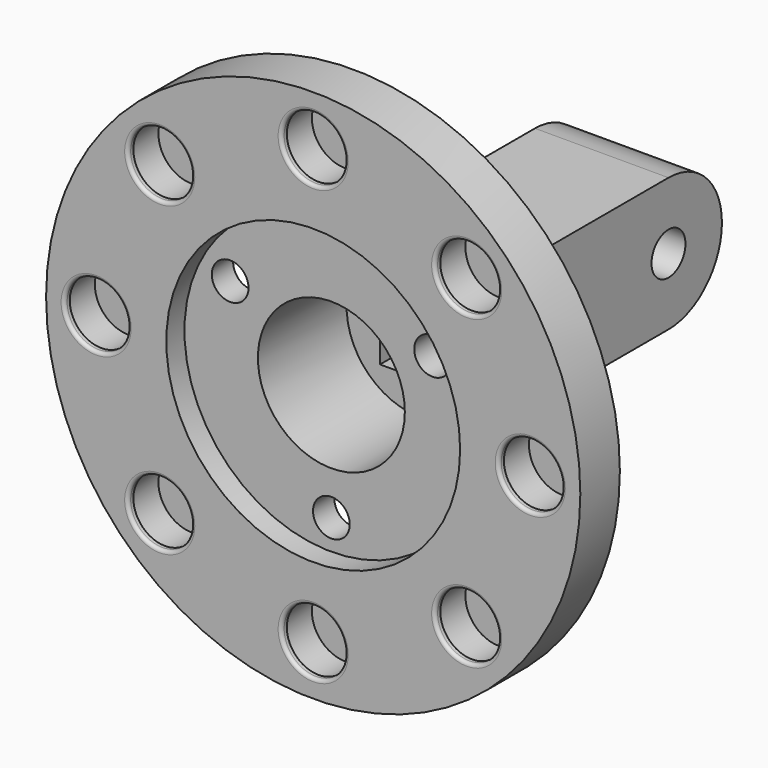
from build123d import *

# Parameters (mm, degrees)
F0_W      = 20
F0_H      = 30
F1_DEPTH  = 20
F2_R      = 9.99999
F3_R      = 3.175
F4_DEPTH  = 25
F5_DEPTH  = 10
F6_T      = -4
F7_R      = 5
F8_DEPTH  = 4
F9_R      = 15
F9_W      = 20
F9_H      = 20
F9_W_2    = 12
F9_H_2    = 12
F10_DEPTH = 4
F11_R     = 15
F11_R_2   = 11
F12_DEPTH = 12.6
F13_R     = 40
F13_R_2   = 15
F13_R_3   = 11
F14_DEPTH = 4
F15_R     = 40
F15_R_2   = 22
F16_DEPTH = 2.4
F17_R     = 2.75
F18_DEPTH = 4
F19_R     = 5
F20_DEPTH = 5
F21_R     = 40
F21_R_2   = 5
F21_R_3   = 22
F21_R_4   = 4.75
F22_DEPTH = 1
F23_R     = 0.5


# Not quite as in the source:
# - a fillet or chamfer is up to 0.001 mm smaller than in the source, because OpenCascade refuses the exact size


with BuildPart() as f1:
    # F0 (on Top) → F1 (new body)
    with BuildSketch(Plane.XY):
        Rectangle(F0_W, F0_H)
    extrude(amount=F1_DEPTH)

    # F2 (radius 10 in the source; OpenCascade refuses exactly that, so slightly less here)
    f2_edges = [f1.edges().sort_by_distance(p)[0] for p in [
        (0, 15, 20),
        (0, 15, 0),
    ]]
    fillet(f2_edges, radius=F2_R)

    # F3 (on face) → F4 (cut)
    with BuildSketch(Plane.YZ.offset(10)):
        with Locations((5, 10)):
            Circle(F3_R)
    extrude(amount=-F4_DEPTH, mode=Mode.SUBTRACT)

    # F5 (add): a face of the model
    f5_faces = [f1.faces().sort_by_distance(p)[0] for p in [
        (0, -15, 10),
    ]]
    extrude(f5_faces, amount=F5_DEPTH)

    # F6
    f6_openings = [f1.faces().sort_by_distance(p)[0] for p in [
        (0, -25, 10),
    ]]
    offset(amount=F6_T, openings=f6_openings)

    # F7 (on face) → F8 (cut)
    with BuildSketch(Plane(origin=(0, 0, 0), x_dir=(1, 0, 0), z_dir=(0, 0, -1))):
        with Locations((0, 10)):
            Circle(F7_R)
    extrude(amount=-F8_DEPTH, mode=Mode.SUBTRACT)

    # F9 (on face) → F10 (join)
    with BuildSketch(Plane.XZ.offset(25)):
        with Locations((0, 10)):
            Circle(F9_R)
        with Locations((0, 10)):
            Rectangle(F9_W, F9_H, mode=Mode.SUBTRACT)
        with Locations((0, 10)):
            Rectangle(F9_W, F9_H)
        with Locations((0, 10)):
            Rectangle(F9_W_2, F9_H_2, mode=Mode.SUBTRACT)
    extrude(amount=F10_DEPTH)

    # F11 (on face) → F12 (join)
    with BuildSketch(Plane.XZ.offset(29)):
        with Locations((0, 10)):
            Circle(F11_R)
        with Locations((0, 10)):
            Circle(F11_R_2, mode=Mode.SUBTRACT)
    extrude(amount=F12_DEPTH)

    # F13 (on face) → F14 (join)
    with BuildSketch(Plane.XZ.offset(41.6)):
        with Locations((0, 10)):
            Circle(F13_R)
        with Locations((0, 10)):
            Circle(F13_R_2, mode=Mode.SUBTRACT)
        with Locations((0, 10)):
            Circle(F13_R_2)
        with Locations((0, 10)):
            Circle(F13_R_3, mode=Mode.SUBTRACT)
    extrude(amount=F14_DEPTH)

    # F15 (on face) → F16 (join)
    with BuildSketch(Plane.XZ.offset(45.6)):
        with Locations((0, 10)):
            Circle(F15_R)
        with Locations((0, 10)):
            Circle(F15_R_2, mode=Mode.SUBTRACT)
    extrude(amount=F16_DEPTH)

    # F17 (on face) → F18 (cut)
    with BuildSketch(Plane.XZ.offset(45.6)):
        with Locations((15.1554445662, 18.75)):
            Circle(F17_R)
        with Locations((0, -7.5)):
            Circle(F17_R)
        with Locations((-15.1554445662, 18.75)):
            Circle(F17_R)
    extrude(amount=-F18_DEPTH, mode=Mode.SUBTRACT)

    # F19 (on face) → F20 (cut)
    with BuildSketch(Plane.XZ.offset(48)):
        with Locations((0, 42.5)):
            Circle(F19_R)
        with Locations((-22.9809703886, 32.9809703886)):
            Circle(F19_R)
        with Locations((-32.5, 10)):
            Circle(F19_R)
        with Locations((-22.9809703886, -12.9809703886)):
            Circle(F19_R)
        with Locations((0, -22.5)):
            Circle(F19_R)
        with Locations((22.9809703886, -12.9809703886)):
            Circle(F19_R)
        with Locations((32.5, 10)):
            Circle(F19_R)
        with Locations((22.9809703886, 32.9809703886)):
            Circle(F19_R)
    extrude(amount=-F20_DEPTH, mode=Mode.SUBTRACT)

    # F21 (on face) → F22 (join)
    with BuildSketch(Plane.XZ.offset(48)):
        with Locations((0, 10)):
            Circle(F21_R)
        with Locations((-22.9809703886, -12.9809703886)):
            Circle(F21_R_2, mode=Mode.SUBTRACT)
        with Locations((0, -22.5)):
            Circle(F21_R_2, mode=Mode.SUBTRACT)
        with Locations((22.9809703886, -12.9809703886)):
            Circle(F21_R_2, mode=Mode.SUBTRACT)
        with Locations((-32.5, 10)):
            Circle(F21_R_2, mode=Mode.SUBTRACT)
        with Locations((-22.9809703886, 32.9809703886)):
            Circle(F21_R_2, mode=Mode.SUBTRACT)
        with Locations((0, 10)):
            Circle(F21_R_3, mode=Mode.SUBTRACT)
        with Locations((32.5, 10)):
            Circle(F21_R_2, mode=Mode.SUBTRACT)
        with Locations((0, 42.5)):
            Circle(F21_R_2, mode=Mode.SUBTRACT)
        with Locations((22.9809703886, 32.9809703886)):
            Circle(F21_R_2, mode=Mode.SUBTRACT)
        with Locations((0, 42.5)):
            Circle(F21_R_2)
        with Locations((0, 42.5)):
            Circle(F21_R_4, mode=Mode.SUBTRACT)
        with Locations((22.9809703886, 32.9809703886)):
            Circle(F21_R_2)
        with Locations((22.9809703886, 32.9809703886)):
            Circle(F21_R_4, mode=Mode.SUBTRACT)
        with Locations((-22.9809703886, 32.9809703886)):
            Circle(F21_R_2)
        with Locations((-22.9809703886, 32.9809703886)):
            Circle(F21_R_4, mode=Mode.SUBTRACT)
        with Locations((32.5, 10)):
            Circle(F21_R_2)
        with Locations((32.5, 10)):
            Circle(F21_R_4, mode=Mode.SUBTRACT)
        with Locations((-32.5, 10)):
            Circle(F21_R_2)
        with Locations((-32.5, 10)):
            Circle(F21_R_4, mode=Mode.SUBTRACT)
        with Locations((-22.9809703886, -12.9809703886)):
            Circle(F21_R_2)
        with Locations((-22.9809703886, -12.9809703886)):
            Circle(F21_R_4, mode=Mode.SUBTRACT)
        with Locations((0, -22.5)):
            Circle(F21_R_2)
        with Locations((0, -22.5)):
            Circle(F21_R_4, mode=Mode.SUBTRACT)
        with Locations((22.9809703886, -12.9809703886)):
            Circle(F21_R_2)
        with Locations((22.9809703886, -12.9809703886)):
            Circle(F21_R_4, mode=Mode.SUBTRACT)
    extrude(amount=F22_DEPTH)

    # F23
    f23_edges = [f1.edges().sort_by_distance(p)[0] for p in [
        (-4.75, -49, 42.5),
        (18.23097, -49, 32.98097),
        (27.75, -49, 10),
        (-27.73097, -49, 32.98097),
        (-37.25, -49, 10),
        (-27.73097, -49, -12.98097),
        (-4.75, -49, -22.5),
        (18.23097, -49, -12.98097),
    ]]
    fillet(f23_edges, radius=F23_R)


solid = f1.part
